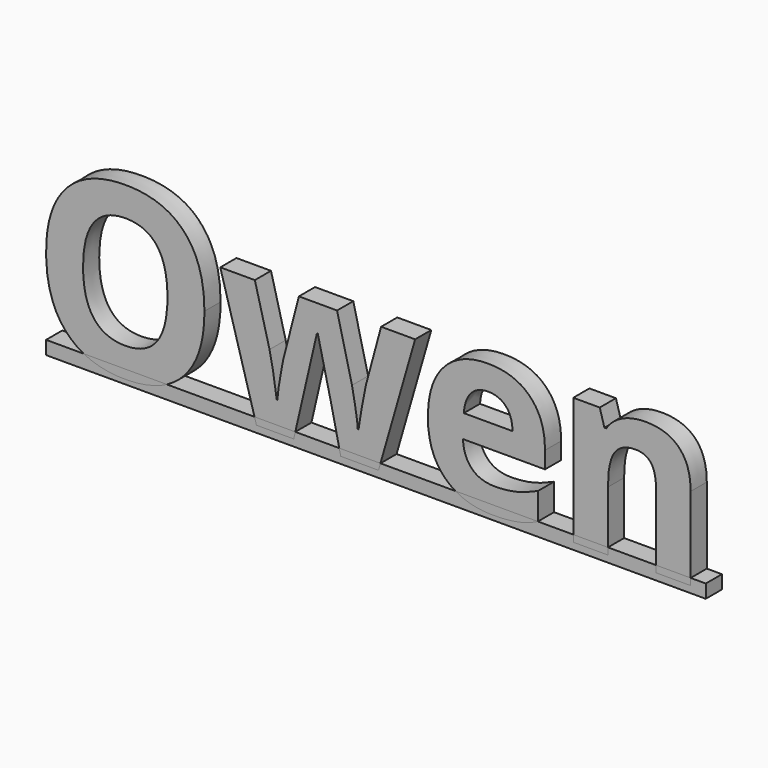
from build123d import *

# Parameters (mm, degrees)
F0_TEXT_SIZE = 34.607689396
F1_DEPTH     = 3
F2_W         = 97.9884280539
F2_H         = 2
F3_DEPTH     = 3


# Not quite as in the source:
# - Text() gives the source's letters only with a copy of the font that has no kerning and outlines rounded to 1/6400 em; it was checked with that copy


with BuildPart() as f1:
    # F0 (on Front) → F1 (new body)
    with BuildSketch(Plane.XZ):
        with Locations((-41.1171755096, 0)):
            Text('Owen', F0_TEXT_SIZE, font='Open Sans', font_style=FontStyle.BOLD, text_align=(TextAlign.LEFT, TextAlign.BOTTOM))
    extrude(amount=F1_DEPTH)

    # F2 (on face) → F3 (join)
    with BuildSketch(Plane.XZ.offset(3)):
        with Locations((9.8886104635, 0)):
            Rectangle(F2_W, F2_H)
    extrude(amount=-F3_DEPTH)


solid = f1.part
